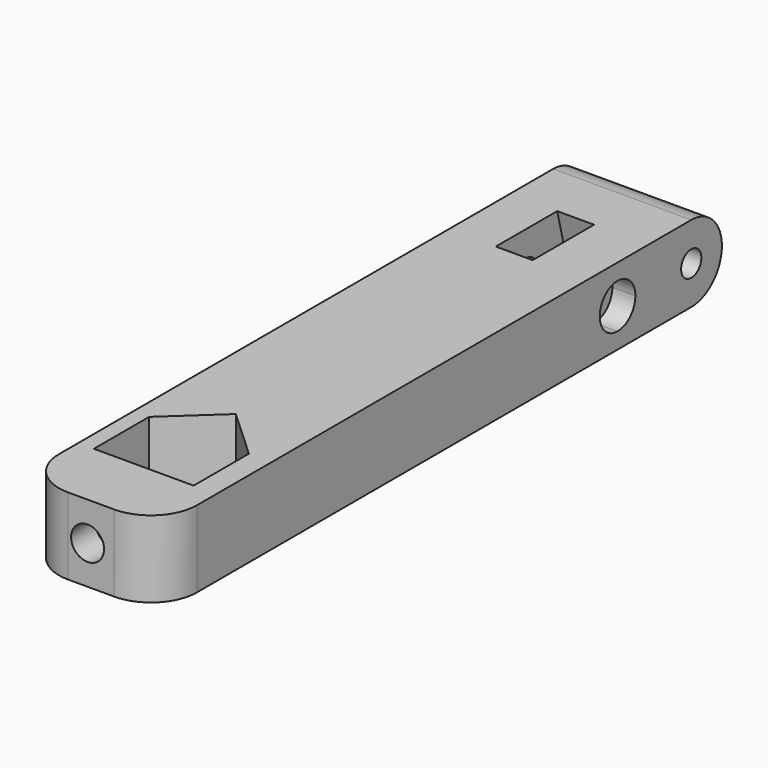
from build123d import *

# Parameters (mm, degrees)
F0_W      = 18
F0_H      = 91.5
F0_W_2    = 7.2
F0_H_2    = 3.15
F0_W_3    = 12
F0_H_3    = 34
F1_DEPTH  = 10
F2_R      = 6
F4_DEPTH  = 7
F5_SIZE   = 2
F6_R      = 1.65
F7_DEPTH  = 25
F8_DEPTH  = 3
F10_R     = 4.99999
F12_DEPTH = 2.4
F15_DEPTH = 2.5
F17_R     = 2.15
F18_DEPTH = 20
F20_W     = 7.2
F20_H     = 3.15
F21_DEPTH = 1.25


# Not quite as in the source:
# - a fillet or chamfer is up to 0.001 mm smaller than in the source, because OpenCascade refuses the exact size


with BuildPart() as f1:
    # F0 (on Top) → F1 (new body)
    with BuildSketch(Plane.XY):
        with Locations((0.4665288143, 11.6095117688)):
            Rectangle(F0_W, F0_H)
        with Locations((0, -28.5654882312)):
            Rectangle(F0_W_2, F0_H_2, mode=Mode.SUBTRACT)
        Polygon((6.5, -24.9904882312), (-6.5, -24.9904882312), (-6.5, -15.9904882312), (0, -9.9904882312), (6.5, -15.9904882312), align=None, mode=Mode.SUBTRACT)
        with Locations((0.4665288143, 11.0095117688)):
            Rectangle(F0_W_3, F0_H_3, mode=Mode.SUBTRACT)
        with Locations((0.4665288143, 11.0095117688)):
            Rectangle(F0_W_3, F0_H_3)
    extrude(amount=F1_DEPTH)

    # F2
    f2_edges = [f1.edges().sort_by_distance(p)[0] for p in [
        (9.466529, -34.140488, 5),
        (-8.533471, -34.140488, 5),
    ]]
    fillet(f2_edges, radius=F2_R)

    # F0 (on Top) → F4 (cut)
    with BuildSketch(Plane.XY):
        with Locations((0.4665288143, 11.0095117688)):
            Rectangle(F0_W_3, F0_H_3)
    extrude(amount=F4_DEPTH, mode=Mode.SUBTRACT)

    # F5
    f5_edges = [f1.edges().sort_by_distance(p)[0] for p in [
        (6.466529, 11.009512, 7),
        (-5.533471, 11.009512, 7),
    ]]
    chamfer(f5_edges, length=F5_SIZE)

    # F6 (on offset) → F7 (cut)
    with BuildSketch(Plane.YZ.offset(9.4665288143)):
        with BuildLine():
            Line((40.3595117688, 3.35), (40.3595117688, 6.65))
            ThreePointArc((40.3595117688, 6.65), (38.7095117688, 5), (40.3595117688, 3.35))
        make_face()
        with BuildLine():
            ThreePointArc((42.0095117688, 5), (41.5262379578, 6.166726189), (40.3595117688, 6.65))
            Line((40.3595117688, 6.65), (40.3595117688, 3.35))
            ThreePointArc((40.3595117688, 3.35), (41.5262379578, 3.833273811), (42.0095117688, 5))
        make_face()
        with Locations((52.3595117688, 5)):
            Circle(F6_R)
    extrude(amount=-F7_DEPTH, mode=Mode.SUBTRACT)

    # F6 (on offset) → F8 (cut)
    with BuildSketch(Plane.YZ.offset(9.4665288143)):
        with BuildLine():
            Line((40.3595117688, 6.65), (40.3595117688, 7.9))
            ThreePointArc((40.3595117688, 7.9), (37.4595117688, 5), (40.3595117688, 2.1))
            Line((40.3595117688, 2.1), (40.3595117688, 3.35))
            ThreePointArc((40.3595117688, 3.35), (38.7095117688, 5), (40.3595117688, 6.65))
        make_face()
        with BuildLine():
            ThreePointArc((43.2595117688, 5), (42.4101214343, 7.0506096654), (40.3595117688, 7.9))
            Line((40.3595117688, 7.9), (40.3595117688, 6.65))
            ThreePointArc((40.3595117688, 6.65), (41.5262379578, 6.166726189), (42.0095117688, 5))
            ThreePointArc((42.0095117688, 5), (41.5262379578, 3.833273811), (40.3595117688, 3.35))
            Line((40.3595117688, 3.35), (40.3595117688, 2.1))
            ThreePointArc((40.3595117688, 2.1), (42.4101214343, 2.9493903346), (43.2595117688, 5))
        make_face()
    extrude(amount=-F8_DEPTH, mode=Mode.SUBTRACT)

    # F10 (radius 5 in the source; OpenCascade refuses exactly that, so slightly less here)
    f10_edges = [f1.edges().sort_by_distance(p)[0] for p in [
        (0.466529, 57.359512, 0),
        (0.466529, 57.359512, 10),
    ]]
    fillet(f10_edges, radius=F10_R)

    # F11 (on offset) → F12 (cut, symmetric)
    with BuildSketch(Plane.YZ):
        Polygon((47.8595117688, 0), (45.3595117688, 10), (35.3595117688, 10), (32.8595117688, 0), align=None)
    extrude(amount=F12_DEPTH, both=True, mode=Mode.SUBTRACT)

    # F14 (on offset) → F15 (cut)
    with BuildSketch(Plane(origin=(-8.5334711857, 0, 0), x_dir=(0, -1, 0), z_dir=(-1, 0, 0))):
        Polygon((-37.5882304767, 3.4), (-37.5882304767, 6.6), (-40.3595117688, 8.2), (-43.1307930609, 6.6), (-43.1307930609, 3.4), (-40.3595117688, 1.8), align=None)
    extrude(amount=-F15_DEPTH, mode=Mode.SUBTRACT)

    # F17 (on offset) → F18 (cut)
    with BuildSketch(Plane.XZ.offset(34.1404882312)):
        with Locations((0, 5)):
            Circle(F17_R)
    extrude(amount=-F18_DEPTH, mode=Mode.SUBTRACT)

    # F20 (on offset) → F21 (join)
    with BuildSketch(Plane.XY.offset(10)):
        with Locations((0, -28.5654882312)):
            Rectangle(F20_W, F20_H)
    extrude(amount=-F21_DEPTH)


solid = f1.part
